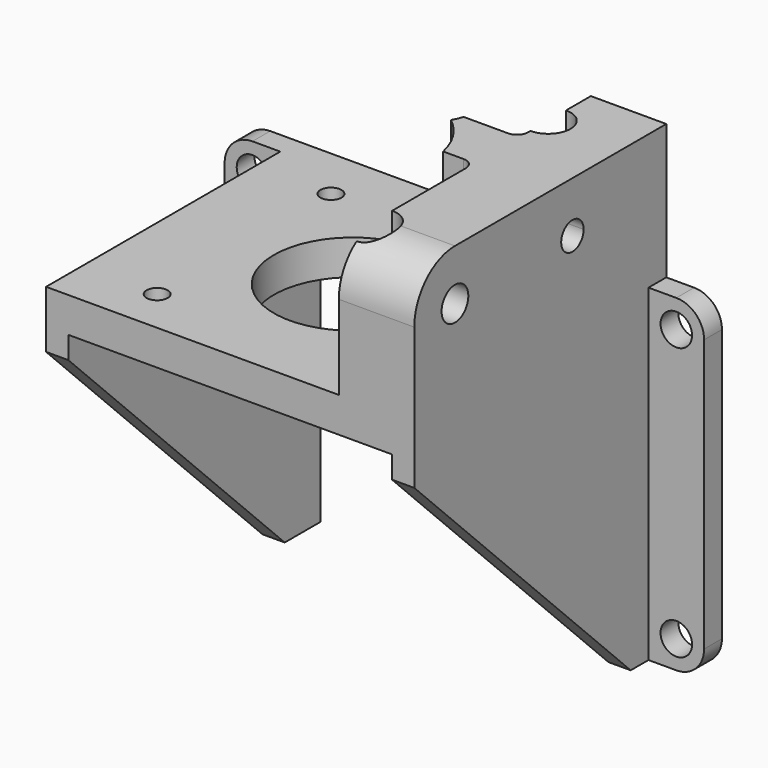
from build123d import *

# Parameters (mm, degrees)
F0_W      = 52.5309846
F0_H      = 44.9404867
F0_R      = 1.5
F0_R_2    = 11.2530001
F1_DEPTH  = 5
F2_W      = 3.175
F2_H      = 44.9404867
F3_DEPTH  = 41.774999
F4_W      = 7.9375
F4_H      = 3.175
F5_DEPTH  = 46.774999
F6_R      = 3.96875
F7_R      = 2.2479
F8_DEPTH  = 3.175
F10_DEPTH = 52.5309846
F12_DEPTH = 19.2659
F14_DEPTH = 10.7654979
F15_R     = 7.9375
F16_DEPTH = 25.4
F17_DEPTH = 30.4370867
F18_R     = 3.175
F19_DEPTH = 19.2659
F21_DEPTH = 133
F22_R     = 7.2517
F23_R     = 1.5875


# Not quite as in the source:
# - an extrude ends at something that could not be found from the text; its depth is read off the source's solid
# - a feature names something its author has since deleted; it is built from what else it names


with BuildPart() as f1:
    # F0 (on Top) → F1 (new body)
    with BuildSketch(Plane.XY):
        with Locations((26.2654923, -22.47024335)):
            Rectangle(F0_W, F0_H)
        with Locations((10.7654979, -38.5904867)):
            Circle(F0_R, mode=Mode.SUBTRACT)
        with Locations((26.2654923, -23.0904923)):
            Circle(F0_R_2, mode=Mode.SUBTRACT)
        with Locations((41.7654867, -38.5904867)):
            Circle(F0_R, mode=Mode.SUBTRACT)
        with Locations((10.7654979, -7.5904979)):
            Circle(F0_R, mode=Mode.SUBTRACT)
        with Locations((41.7654867, -7.5904979)):
            Circle(F0_R, mode=Mode.SUBTRACT)
    extrude(amount=F1_DEPTH)

    # F2 (on face) → F3 (join)
    with BuildSketch(Plane(origin=(0, 0, 0), x_dir=(1, 0, 0), z_dir=(0, 0, -1))):
        with Locations((1.5875, 22.47024335)):
            Rectangle(F2_W, F2_H)
        with Locations((50.9434846, 22.47024335)):
            Rectangle(F2_W, F2_H)
    extrude(amount=F3_DEPTH)

    # F4 (on face) → F5 (join, through all)
    with BuildSketch(Plane(origin=(0, 0, -41.774999), x_dir=(1, 0, 0), z_dir=(0, 0, -1))):
        with Locations((-3.96875, 1.5875)):
            Rectangle(F4_W, F4_H)
        with Locations((56.4997346, 1.5875)):
            Rectangle(F4_W, F4_H)
    extrude(amount=-F5_DEPTH)

    # F6
    f6_edges = [f1.edges().sort_by_distance(p)[0] for p in [
        (60.468485, -1.5875, -41.774999),
        (60.468485, -1.5875, 5),
        (-7.9375, -1.5875, 5),
        (-7.9375, -1.5875, -41.774999),
    ]]
    fillet(f6_edges, radius=F6_R)

    # F7 (on face) → F8 (cut, through all)
    with BuildSketch(Plane(origin=(0, 0, 0), x_dir=(-1, 0, 0), z_dir=(0, 1, 0))):
        with Locations((3.96875, -37.806249)):
            Circle(F7_R)
        with Locations((3.96875, 1.03125)):
            Circle(F7_R)
        with Locations((-56.4997346, 1.03125)):
            Circle(F7_R)
        with Locations((-56.4997346, -37.806249)):
            Circle(F7_R)
    extrude(amount=-F8_DEPTH, mode=Mode.SUBTRACT)

    # F9 (on face) → F10 (cut, through all)
    with BuildSketch(Plane.YZ.offset(52.5309846)):
        Polygon((-44.9404867, -3.175), (-44.9404867, -41.774999), (-6.35, -41.774999), align=None)
    extrude(amount=-F10_DEPTH, mode=Mode.SUBTRACT)

    # F11 (on face) → F12 (join)
    with BuildSketch(Plane.XY.offset(5)):
        with BuildLine():
            Line((41.7654867, -44.9404867), (52.5309846, -44.9404867))
            Line((52.5309846, -44.9404867), (52.5309846, -30.4370867))
            Line((52.5309846, -30.4370867), (41.7654867, -30.4370867))
            Line((41.7654867, -30.4370867), (41.7654867, -35.4154867))
            ThreePointArc((41.7654867, -35.4154867), (44.9404867, -38.5904867), (41.7654867, -41.7654867))
            Line((41.7654867, -41.7654867), (41.7654867, -44.9404867))
        make_face()
        with BuildLine():
            Line((52.5309846, -20.7092423), (52.5309846, -12.7717423))
            Line((52.5309846, -12.7717423), (30.7547472146, -12.7717423))
            ThreePointArc((30.7547472146, -12.7717423), (34.966988133, -15.9550889113), (37.2636584966, -20.7092423))
            Line((37.2636584966, -20.7092423), (52.5309846, -20.7092423))
        make_face()
    extrude(amount=F12_DEPTH)

    # F13 (on face) → F14 (cut, through all)
    with BuildSketch(Plane.YZ.offset(52.5309846)):
        with BuildLine():
            Line((-40.0700367, 17.0142), (-37.6887867, 17.0142))
            Line((-37.6887867, 17.0142), (-37.6887867, 14.63295))
            ThreePointArc((-37.6887867, 14.63295), (-36.0049886773, 15.3304019773), (-35.3075367, 17.0142))
            ThreePointArc((-35.3075367, 17.0142), (-37.6887867, 19.39545), (-40.0700367, 17.0142))
        make_face()
        with BuildLine():
            Line((-37.6887867, 14.63295), (-37.6887867, 17.0142))
            Line((-37.6887867, 17.0142), (-40.0700367, 17.0142))
            ThreePointArc((-40.0700367, 17.0142), (-39.3725847227, 15.3304019773), (-37.6887867, 14.63295))
        make_face()
    extrude(amount=-F14_DEPTH, mode=Mode.SUBTRACT)

    # F15 (on face) → F16 (cut)
    with BuildSketch(Plane.XY.offset(5)):
        with Locations((26.2654923, -10.3904923)):
            Circle(F15_R)
    extrude(amount=F16_DEPTH, mode=Mode.SUBTRACT)

    # F17 (add, through all): a face of the model
    f17_faces = [f1.faces().sort_by_distance(p)[0] for p in [
        (47.14823565, -30.4370867, 14.63295),
    ]]
    extrude(f17_faces, amount=F17_DEPTH)

    # F18 (on face) → F19 (cut, through all)
    with BuildSketch(Plane.XY.offset(5)):
        with Locations((41.7654867, -7.5904979)):
            Circle(F18_R)
    extrude(amount=F19_DEPTH, mode=Mode.SUBTRACT)

    # F20 (on face) → F21 (cut, through all)
    with BuildSketch(Plane.YZ.offset(52.5309846)):
        with BuildLine():
            ThreePointArc((-16.7404923, 19.0142), (-18.1547058624, 18.4284135624), (-18.7404923, 17.0142))
            Line((-18.7404923, 17.0142), (-16.7404923, 17.0142))
            Line((-16.7404923, 17.0142), (-16.7404923, 19.0142))
        make_face()
        with BuildLine():
            Line((-16.7404923, 17.0142), (-18.7404923, 17.0142))
            ThreePointArc((-18.7404923, 17.0142), (-16.7404923, 15.0142), (-14.7404923, 17.0142))
            ThreePointArc((-14.7404923, 17.0142), (-15.3262787376, 18.4284135624), (-16.7404923, 19.0142))
            Line((-16.7404923, 19.0142), (-16.7404923, 17.0142))
        make_face()
    extrude(amount=-F21_DEPTH, mode=Mode.SUBTRACT)

    # F22
    f22_edges = [f1.edges().sort_by_distance(p)[0] for p in [
        (47.148236, -44.940487, 24.2659),
    ]]
    fillet(f22_edges, radius=F22_R)

    # F23
    f23_edges = [f1.edges().sort_by_distance(p)[0] for p in [
        (41.765487, -20.709242, 14.63295),
        (41.765487, -12.771742, 14.63295),
    ]]
    fillet(f23_edges, radius=F23_R)


solid = f1.part
